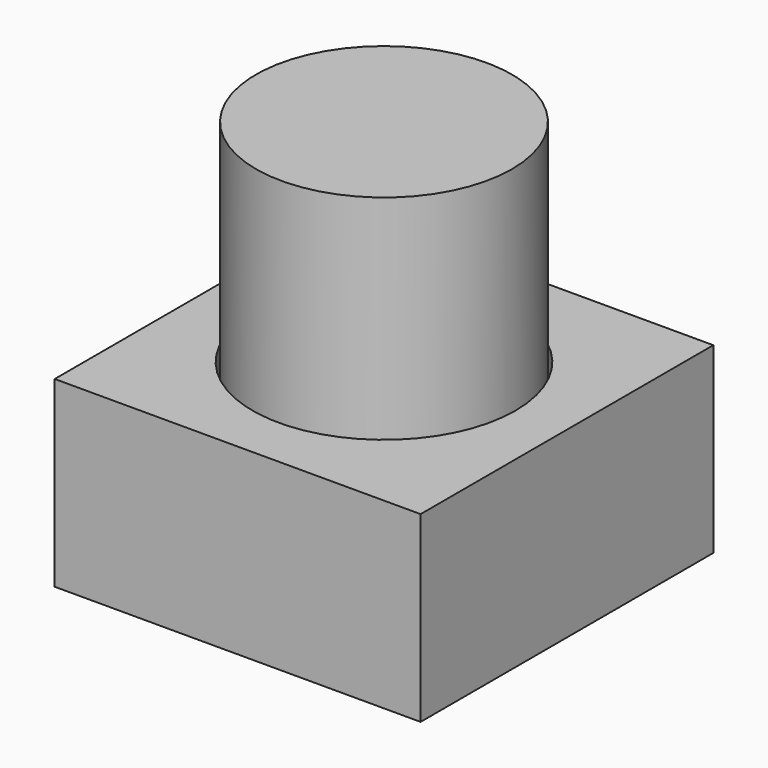
from build123d import *

# Parameters (mm, degrees)
F0_W      = 64
F0_H      = 64
F1_DEPTH  = 32
F2_R      = 23
F3_DEPTH  = 25
F5_R      = 22.4
F6_DEPTH  = 62
F8_START  = -15
F7_R      = 14.1
F8_DEPTH  = 22.8
F10_START = 1.2
F9_W      = 5
F9_H      = 86.7077708244
F10_DEPTH = 23.8
F11_R     = 2.4999
F13_DEPTH = 10
F15_DEPTH = 10


# Not quite as in the source:
# - a fillet or chamfer is up to 0.001 mm smaller than in the source, because OpenCascade refuses the exact size


with BuildPart() as f1:
    # F0 (on Top) → F1 (new body)
    with BuildSketch(Plane.XY):
        Rectangle(F0_W, F0_H)
    extrude(amount=F1_DEPTH)

    # F2 (on face) → F3 (cut)
    with BuildSketch(Plane.XY.offset(32)):
        Circle(F2_R)
    extrude(amount=-F3_DEPTH, mode=Mode.SUBTRACT)

    # F14 (on face) → F15 (join)
    with BuildSketch(Plane.XY.offset(7)):
        Polygon((5.1776695297, 12.5), (-5.1776695297, 12.5), (-12.5, 5.1776695297), (-12.5, -5.1776695297), (-5.1776695297, -12.5), (5.1776695297, -12.5), (12.5, -5.1776695297), (12.5, 5.1776695297), align=None)
    extrude(amount=F15_DEPTH)


with BuildPart() as f6:
    # F5 (on face) → F6 (new body)
    with BuildSketch(Plane.XY.offset(7)):
        Circle(F5_R)
    extrude(amount=F6_DEPTH)

    # F7 (on Right) → F8 (cut)
    with BuildSketch(Plane.YZ.offset(F8_START)):
        with Locations((0, 52.1)):
            Circle(F7_R)
    extrude(amount=-F8_DEPTH, mode=Mode.SUBTRACT)

    # F9 (on face) → F10 (cut)
    with BuildSketch(Plane(origin=(-15, 0, 0), x_dir=(0, -1, 0), z_dir=(-1, 0, 0)).offset(F10_START)):
        Rectangle(F9_W, F9_H)
    extrude(amount=F10_DEPTH, mode=Mode.SUBTRACT)

    # F11 (radius 2.5 in the source; OpenCascade refuses exactly that, so slightly less here)
    f11_edges = [f6.edges().sort_by_distance(p)[0] for p in [
        (-16.2, 2.5, 22.6117),
        (-16.2, -2.5, 22.6117),
    ]]
    fillet(f11_edges, radius=F11_R)

    # F12 (on face) → F13 (cut)
    with BuildSketch(Plane.XY.offset(7)):
        Polygon((11, -4.5563491861), (11, 4.5563491861), (4.5563491861, 11), (-4.5563491861, 11), (-11, 4.5563491861), (-11, -4.5563491861), (-4.5563491861, -11), (4.5563491861, -11), align=None)
    extrude(amount=F13_DEPTH, mode=Mode.SUBTRACT)


solid = Compound([f1.part, f6.part])
